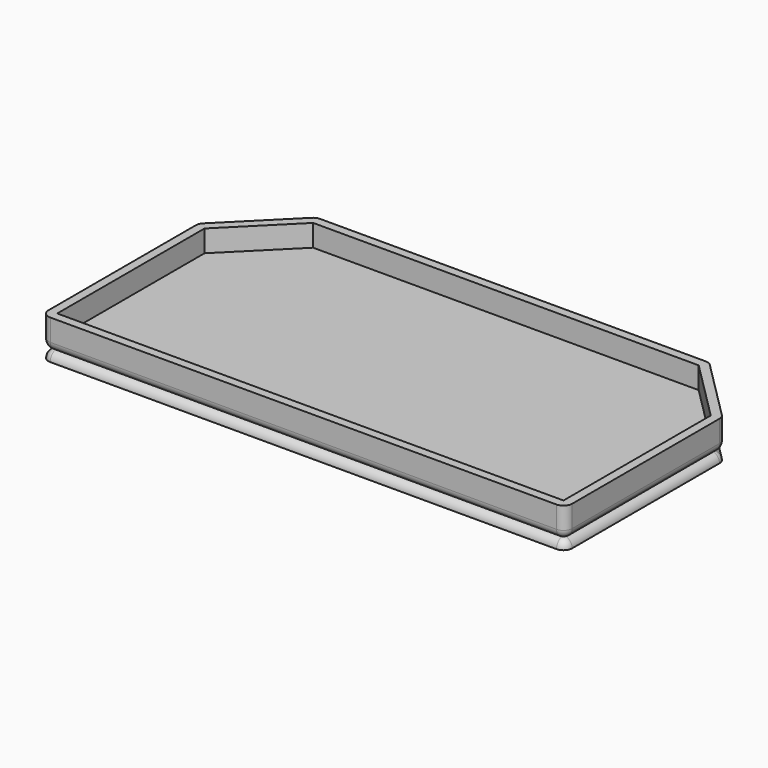
from build123d import *

# Parameters (mm, degrees)
F1_DEPTH = 2
F2_R     = 1.99999
F4_DEPTH = 5
F5_DEPTH = 2
F6_R     = 1.99999


# Not quite as in the source:
# - a fillet or chamfer is up to 0.001 mm smaller than in the source, because OpenCascade refuses the exact size


with BuildPart() as f1:
    # F0 (on Top) → F1 (new body)
    with BuildSketch(Plane.XY):
        with BuildLine():
            ThreePointArc((-60, -28), (-59.4142135624, -29.4142135624), (-58, -30))
            Line((-58, -30), (58, -30))
            ThreePointArc((58, -30), (59.4142135624, -29.4142135624), (60, -28))
            Line((60, -28), (60, 14.1715728753))
            ThreePointArc((60, 14.1715728753), (59.847759065, 14.93693974), (59.4142135624, 15.5857864376))
            Line((59.4142135624, 15.5857864376), (45.5857864376, 29.4142135624))
            ThreePointArc((45.5857864376, 29.4142135624), (44.93693974, 29.847759065), (44.1715728753, 30))
            Line((44.1715728753, 30), (-44.1715728753, 30))
            ThreePointArc((-44.1715728753, 30), (-44.93693974, 29.847759065), (-45.5857864376, 29.4142135624))
            Line((-45.5857864376, 29.4142135624), (-59.4142135624, 15.5857864376))
            ThreePointArc((-59.4142135624, 15.5857864376), (-59.847759065, 14.93693974), (-60, 14.1715728753))
            Line((-60, 14.1715728753), (-60, -28))
        make_face()
    extrude(amount=F1_DEPTH)

    # F2 (radius 2 in the source; OpenCascade refuses exactly that, so slightly less here)
    f2_edges = [f1.edges().sort_by_distance(p)[0] for p in [
        (0, -30, 0),
        (-60, -6.914214, 0),
        (0, 30, 0),
        (52.5, 22.5, 0),
        (60, -6.914214, 0),
        (-52.5, 22.5, 0),
    ]]
    fillet(f2_edges, radius=F2_R)

    # F3 (on face) → F4 (join)
    with BuildSketch(Plane.XY.offset(2)):
        with BuildLine():
            Line((-45.5857864376, 29.4142135624), (-59.4142135624, 15.5857864376))
            ThreePointArc((-59.4142135624, 15.5857864376), (-59.847759065, 14.93693974), (-60, 14.1715728753))
            Line((-60, 14.1715728753), (-60, -28))
            ThreePointArc((-60, -28), (-59.4142135624, -29.4142135624), (-58, -30))
            Line((-58, -30), (58, -30))
            ThreePointArc((58, -30), (59.4142135624, -29.4142135624), (60, -28))
            Line((60, -28), (60, 14.1715728753))
            ThreePointArc((60, 14.1715728753), (59.847759065, 14.93693974), (59.4142135624, 15.5857864376))
            Line((59.4142135624, 15.5857864376), (45.5857864376, 29.4142135624))
            ThreePointArc((45.5857864376, 29.4142135624), (44.93693974, 29.847759065), (44.1715728753, 30))
            Line((44.1715728753, 30), (-44.1715728753, 30))
            ThreePointArc((-44.1715728753, 30), (-44.93693974, 29.847759065), (-45.5857864376, 29.4142135624))
        make_face()
        Polygon((-44.1715728753, 28), (44.1715728753, 28), (58, 14.1715728753), (58, -28), (-58, -28), (-58, 14.1715728753), align=None, mode=Mode.SUBTRACT)
    extrude(amount=F4_DEPTH)


with BuildPart() as f5:
    # F0 (on Top) → F5 (new body)
    with BuildSketch(Plane.XY):
        with BuildLine():
            ThreePointArc((-60, -28), (-59.4142135624, -29.4142135624), (-58, -30))
            Line((-58, -30), (58, -30))
            ThreePointArc((58, -30), (59.4142135624, -29.4142135624), (60, -28))
            Line((60, -28), (60, 14.1715728753))
            ThreePointArc((60, 14.1715728753), (59.847759065, 14.93693974), (59.4142135624, 15.5857864376))
            Line((59.4142135624, 15.5857864376), (45.5857864376, 29.4142135624))
            ThreePointArc((45.5857864376, 29.4142135624), (44.93693974, 29.847759065), (44.1715728753, 30))
            Line((44.1715728753, 30), (-44.1715728753, 30))
            ThreePointArc((-44.1715728753, 30), (-44.93693974, 29.847759065), (-45.5857864376, 29.4142135624))
            Line((-45.5857864376, 29.4142135624), (-59.4142135624, 15.5857864376))
            ThreePointArc((-59.4142135624, 15.5857864376), (-59.847759065, 14.93693974), (-60, 14.1715728753))
            Line((-60, 14.1715728753), (-60, -28))
        make_face()
    extrude(amount=-F5_DEPTH)

    # F6 (radius 2 in the source; OpenCascade refuses exactly that, so slightly less here)
    f6_edges = [f5.edges().sort_by_distance(p)[0] for p in [
        (-60, -6.914214, 0),
    ]]
    fillet(f6_edges, radius=F6_R)


solid = Compound([f1.part, f5.part])
